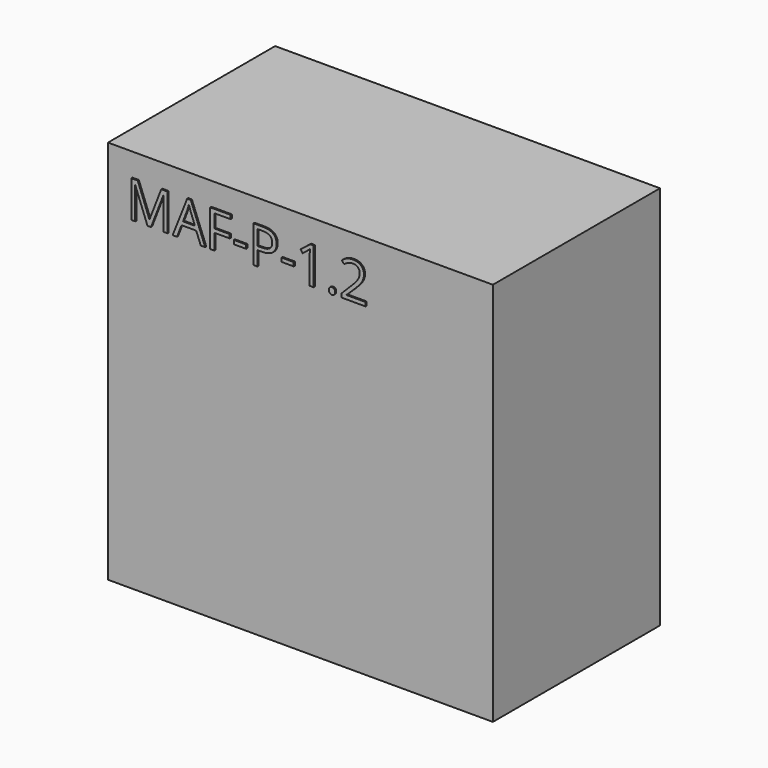
from build123d import *

# Parameters (mm, degrees)
F0_W         = 1778
F0_H         = 711.2
F1_DEPTH     = 1778
F2_TEXT_SIZE = 237.5442120764
F3_DEPTH     = 6.35
F4_DEPTH     = 254


# Not quite as in the source:
# - Text() gives the source's letters only with a copy of the font that has no kerning and outlines rounded to 1/6400 em; it was checked with that copy


with BuildPart() as f1:
    # F0 (on Top) → F1 (new body)
    with BuildSketch(Plane.XY):
        with Locations((889, 355.6)):
            Rectangle(F0_W, F0_H)
    extrude(amount=F1_DEPTH)

    # F2 (on face) → F3 (join)
    with BuildSketch(Plane.XZ):
        with Locations((89.3851667643, 1502.6346445084)):
            Text('MAF-P-1.2', F2_TEXT_SIZE, font='Open Sans', text_align=(TextAlign.LEFT, TextAlign.BOTTOM))
    extrude(amount=F3_DEPTH)

    # F4 (add): a face of the model
    f4_faces = [f1.faces().sort_by_distance(p)[0] for p in [
        (889, 711.2, 889),
    ]]
    extrude(f4_faces, amount=F4_DEPTH)


solid = f1.part
